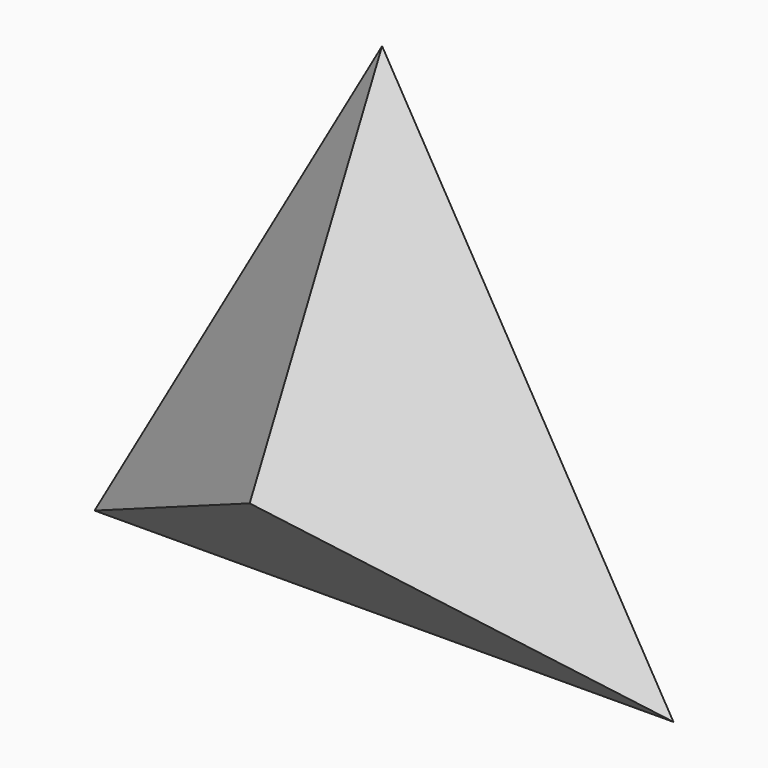
from build123d import *


# Not quite as in the source:
# - an extrude whose draft closes it to a point is written as a loft to that point


with BuildPart() as f1:
    # F0 (on Front) → F1 section 0
    with BuildSketch(Plane.XZ, mode=Mode.PRIVATE) as f1_s0:
        Polygon((-0.2789320431, 73.3229536383), (-63.3600745098, -36.9030390544), (63.6390065529, -36.4199145839), align=None)
    loft([f1_s0.sketch, Vertex(0, -36.6617420935, 0)], ruled=True)


solid = f1.part
